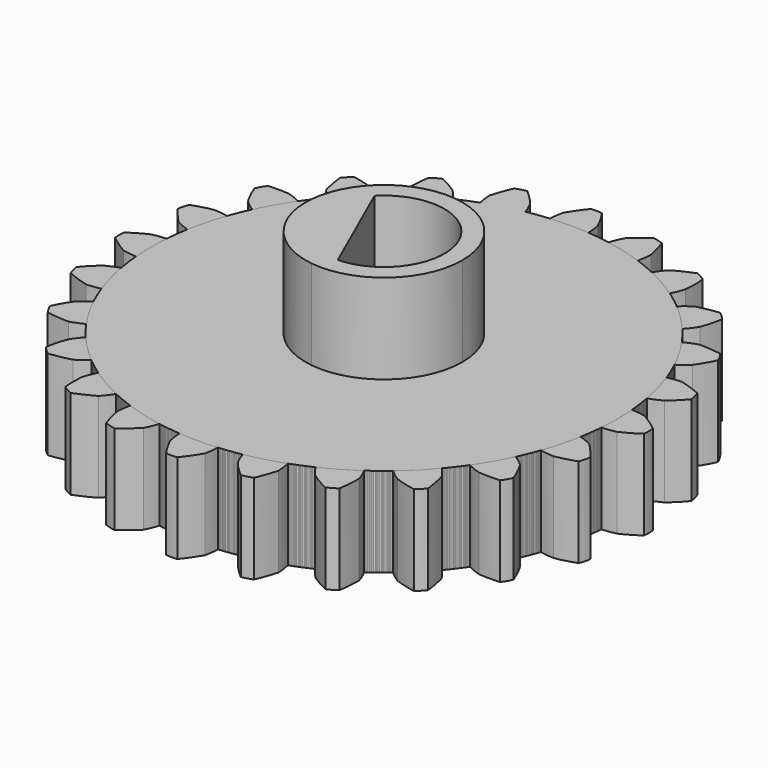
from build123d import *

# Parameters (mm, degrees)
F1_DEPTH = 5
F2_COUNT = 24
F4_DEPTH = 25
F6_DEPTH = 5


# Not quite as in the source:
# - a feature names something its author has since deleted; it is built from what else it names


with BuildPart() as f1:
    # F0 (on Top) → F1 (new body)
    with BuildSketch(Plane.XY):
        with BuildLine():
            ThreePointArc((-1.0909404477, 13.2232983115), (-8.7845379641, -9.3037195236), (13.009999547, 0.2700002324))
            ThreePointArc((13.009999547, 0.2700002324), (9.5634676777, 9.0865328091), (1.0513462123, 13.2282253085))
            ThreePointArc((1.0513462123, 13.2282253085), (-0.0198987816, 13.2699658512), (-1.0909404477, 13.2232983115))
        make_face()
        with BuildLine():
            ThreePointArc((-1.0909404477, 13.2232983115), (-0.0198987816, 13.2699658512), (1.0513462123, 13.2282253085))
            ThreePointArc((1.0513462123, 13.2282253085), (1.0154705709, 13.6241870699), (0.9417103543, 14.0148687927))
            ThreePointArc((0.9417103543, 14.0148687927), (0.6685218353, 14.5430546668), (0.3473408595, 15.0435095252))
            ThreePointArc((0.3473408595, 15.0435095252), (0.03481123, 15.0619613653), (-0.2776888118, 15.0430150292))
            ThreePointArc((-0.2776888118, 15.0430150292), (-0.6507511868, 14.5395305502), (-0.9878320882, 14.0112800205))
            ThreePointArc((-0.9878320882, 14.0112800205), (-1.0583416545, 13.6197695013), (-1.0909404477, 13.2232983115))
        make_face()
    extrude(amount=F1_DEPTH)


with BuildPart() as f2_1:
    # F2: instance of F1
    add(f1.part.rotate(Axis((0.009999547, 0.2700002324, 0), (0, 0, -1)), 1 * 360 / F2_COUNT))


with BuildPart() as f2_2:
    # F2: instance of F1
    add(f1.part.rotate(Axis((0.009999547, 0.2700002324, 0), (0, 0, -1)), 2 * 360 / F2_COUNT))


with BuildPart() as f2_3:
    # F2: instance of F1
    add(f1.part.rotate(Axis((0.009999547, 0.2700002324, 0), (0, 0, -1)), 3 * 360 / F2_COUNT))


with BuildPart() as f2_4:
    # F2: instance of F1
    add(f1.part.rotate(Axis((0.009999547, 0.2700002324, 0), (0, 0, -1)), 4 * 360 / F2_COUNT))


with BuildPart() as f2_5:
    # F2: instance of F1
    add(f1.part.rotate(Axis((0.009999547, 0.2700002324, 0), (0, 0, -1)), 5 * 360 / F2_COUNT))


with BuildPart() as f2_6:
    # F2: instance of F1
    add(f1.part.rotate(Axis((0.009999547, 0.2700002324, 0), (0, 0, -1)), 6 * 360 / F2_COUNT))


with BuildPart() as f2_7:
    # F2: instance of F1
    add(f1.part.rotate(Axis((0.009999547, 0.2700002324, 0), (0, 0, -1)), 7 * 360 / F2_COUNT))


with BuildPart() as f2_8:
    # F2: instance of F1
    add(f1.part.rotate(Axis((0.009999547, 0.2700002324, 0), (0, 0, -1)), 8 * 360 / F2_COUNT))


with BuildPart() as f2_9:
    # F2: instance of F1
    add(f1.part.rotate(Axis((0.009999547, 0.2700002324, 0), (0, 0, -1)), 9 * 360 / F2_COUNT))


with BuildPart() as f2_10:
    # F2: instance of F1
    add(f1.part.rotate(Axis((0.009999547, 0.2700002324, 0), (0, 0, -1)), 10 * 360 / F2_COUNT))


with BuildPart() as f2_11:
    # F2: instance of F1
    add(f1.part.rotate(Axis((0.009999547, 0.2700002324, 0), (0, 0, -1)), 11 * 360 / F2_COUNT))


with BuildPart() as f2_12:
    # F2: instance of F1
    add(f1.part.rotate(Axis((0.009999547, 0.2700002324, 0), (0, 0, -1)), 12 * 360 / F2_COUNT))


with BuildPart() as f2_13:
    # F2: instance of F1
    add(f1.part.rotate(Axis((0.009999547, 0.2700002324, 0), (0, 0, -1)), 13 * 360 / F2_COUNT))


with BuildPart() as f2_14:
    # F2: instance of F1
    add(f1.part.rotate(Axis((0.009999547, 0.2700002324, 0), (0, 0, -1)), 14 * 360 / F2_COUNT))


with BuildPart() as f2_15:
    # F2: instance of F1
    add(f1.part.rotate(Axis((0.009999547, 0.2700002324, 0), (0, 0, -1)), 15 * 360 / F2_COUNT))


with BuildPart() as f2_16:
    # F2: instance of F1
    add(f1.part.rotate(Axis((0.009999547, 0.2700002324, 0), (0, 0, -1)), 16 * 360 / F2_COUNT))


with BuildPart() as f2_17:
    # F2: instance of F1
    add(f1.part.rotate(Axis((0.009999547, 0.2700002324, 0), (0, 0, -1)), 17 * 360 / F2_COUNT))


with BuildPart() as f2_18:
    # F2: instance of F1
    add(f1.part.rotate(Axis((0.009999547, 0.2700002324, 0), (0, 0, -1)), 18 * 360 / F2_COUNT))


with BuildPart() as f2_19:
    # F2: instance of F1
    add(f1.part.rotate(Axis((0.009999547, 0.2700002324, 0), (0, 0, -1)), 19 * 360 / F2_COUNT))


with BuildPart() as f2_20:
    # F2: instance of F1
    add(f1.part.rotate(Axis((0.009999547, 0.2700002324, 0), (0, 0, -1)), 20 * 360 / F2_COUNT))


with BuildPart() as f2_21:
    # F2: instance of F1
    add(f1.part.rotate(Axis((0.009999547, 0.2700002324, 0), (0, 0, -1)), 21 * 360 / F2_COUNT))


with BuildPart() as f2_22:
    # F2: instance of F1
    add(f1.part.rotate(Axis((0.009999547, 0.2700002324, 0), (0, 0, -1)), 22 * 360 / F2_COUNT))


with BuildPart() as f2_23:
    # F2: instance of F1
    add(f1.part.rotate(Axis((0.009999547, 0.2700002324, 0), (0, 0, -1)), 23 * 360 / F2_COUNT))


with BuildPart() as f4_tool:
    # F3 (on face) → F4 (new body)
    with BuildSketch(Plane.XY.offset(5)):
        with BuildLine():
            ThreePointArc((0.133673408, -3.1189176238), (2.4512552702, -2.0837903178), (3.4011733055, 0.2700002324))
            ThreePointArc((3.4011733055, 0.2700002324), (2.404383524, 2.6714549646), (0, 3.661159248))
            ThreePointArc((0, 3.661159248), (-1.3078927109, 3.3946153217), (-2.4116129926, 2.6439952129))
            Line((-2.4116129926, 2.6439952129), (0.133673408, -3.1189176238))
        make_face()
    extrude(amount=-F4_DEPTH)


with BuildPart() as f1_1:
    add(f1.part)

    # F4: cut by f4_tool
    add(f4_tool.part, mode=Mode.SUBTRACT)


with BuildPart() as f2_1_1:
    add(f2_1.part)

    # F4: cut by f4_tool
    add(f4_tool.part, mode=Mode.SUBTRACT)


with BuildPart() as f2_2_1:
    add(f2_2.part)

    # F4: cut by f4_tool
    add(f4_tool.part, mode=Mode.SUBTRACT)


with BuildPart() as f2_3_1:
    add(f2_3.part)

    # F4: cut by f4_tool
    add(f4_tool.part, mode=Mode.SUBTRACT)


with BuildPart() as f2_4_1:
    add(f2_4.part)

    # F4: cut by f4_tool
    add(f4_tool.part, mode=Mode.SUBTRACT)


with BuildPart() as f2_5_1:
    add(f2_5.part)

    # F4: cut by f4_tool
    add(f4_tool.part, mode=Mode.SUBTRACT)


with BuildPart() as f2_6_1:
    add(f2_6.part)

    # F4: cut by f4_tool
    add(f4_tool.part, mode=Mode.SUBTRACT)


with BuildPart() as f2_7_1:
    add(f2_7.part)

    # F4: cut by f4_tool
    add(f4_tool.part, mode=Mode.SUBTRACT)


with BuildPart() as f2_8_1:
    add(f2_8.part)

    # F4: cut by f4_tool
    add(f4_tool.part, mode=Mode.SUBTRACT)


with BuildPart() as f2_9_1:
    add(f2_9.part)

    # F4: cut by f4_tool
    add(f4_tool.part, mode=Mode.SUBTRACT)


with BuildPart() as f2_10_1:
    add(f2_10.part)

    # F4: cut by f4_tool
    add(f4_tool.part, mode=Mode.SUBTRACT)


with BuildPart() as f2_11_1:
    add(f2_11.part)

    # F4: cut by f4_tool
    add(f4_tool.part, mode=Mode.SUBTRACT)


with BuildPart() as f2_12_1:
    add(f2_12.part)

    # F4: cut by f4_tool
    add(f4_tool.part, mode=Mode.SUBTRACT)


with BuildPart() as f2_13_1:
    add(f2_13.part)

    # F4: cut by f4_tool
    add(f4_tool.part, mode=Mode.SUBTRACT)


with BuildPart() as f2_14_1:
    add(f2_14.part)

    # F4: cut by f4_tool
    add(f4_tool.part, mode=Mode.SUBTRACT)


with BuildPart() as f2_15_1:
    add(f2_15.part)

    # F4: cut by f4_tool
    add(f4_tool.part, mode=Mode.SUBTRACT)


with BuildPart() as f2_16_1:
    add(f2_16.part)

    # F4: cut by f4_tool
    add(f4_tool.part, mode=Mode.SUBTRACT)


with BuildPart() as f2_17_1:
    add(f2_17.part)

    # F4: cut by f4_tool
    add(f4_tool.part, mode=Mode.SUBTRACT)


with BuildPart() as f2_18_1:
    add(f2_18.part)

    # F4: cut by f4_tool
    add(f4_tool.part, mode=Mode.SUBTRACT)


with BuildPart() as f2_19_1:
    add(f2_19.part)

    # F4: cut by f4_tool
    add(f4_tool.part, mode=Mode.SUBTRACT)


with BuildPart() as f2_20_1:
    add(f2_20.part)

    # F4: cut by f4_tool
    add(f4_tool.part, mode=Mode.SUBTRACT)


with BuildPart() as f2_21_1:
    add(f2_21.part)

    # F4: cut by f4_tool
    add(f4_tool.part, mode=Mode.SUBTRACT)


with BuildPart() as f2_22_1:
    add(f2_22.part)

    # F4: cut by f4_tool
    add(f4_tool.part, mode=Mode.SUBTRACT)


with BuildPart() as f2_23_1:
    add(f2_23.part)

    # F4: cut by f4_tool
    add(f4_tool.part, mode=Mode.SUBTRACT)


with BuildPart() as f6:
    # F5 (on face) → F6 (new body)
    with BuildSketch(Plane.XY.offset(5)):
        with BuildLine():
            ThreePointArc((-3.1464370209, 1.4647944375), (0.6173098397, 3.5899097505), (3.384999547, 0.2700002324))
            ThreePointArc((3.384999547, 0.2700002324), (1.9589480435, -2.4853989688), (-1.1140966058, -2.9122996968))
            Line((-1.1140966058, -2.9122996968), (-0.5787908965, -4.0651988188))
            ThreePointArc((-0.5787908965, -4.0651988188), (2.8879038896, -3.0251919616), (4.384999547, 0.2700002324))
            ThreePointArc((4.384999547, 0.2700002324), (1.2325486334, 4.4707143064), (-3.6817427302, 2.6176935595))
            Line((-3.6817427302, 2.6176935595), (-3.1464370209, 1.4647944375))
        make_face()
        with BuildLine():
            ThreePointArc((-1.1140966058, -2.9122996968), (-3.0511241614, -1.1513183954), (-3.1464370209, 1.4647944375))
            Line((-3.1464370209, 1.4647944375), (-3.6817427302, 2.6176935595))
            ThreePointArc((-3.6817427302, 2.6176935595), (-3.9581237787, -1.5724498406), (-0.5787908965, -4.0651988188))
            Line((-0.5787908965, -4.0651988188), (-1.1140966058, -2.9122996968))
        make_face()
        with BuildLine():
            Line((0.1266359476, -3.1029837507), (-2.4045755323, 2.6280613398))
            ThreePointArc((-2.4045755323, 2.6280613398), (-2.8355830234, 2.0847412153), (-3.1464370209, 1.4647944375))
            Line((-3.1464370209, 1.4647944375), (-1.1140966058, -2.9122996968))
            ThreePointArc((-1.1140966058, -2.9122996968), (-0.5026737312, -3.0658341625), (0.1266359476, -3.1029837507))
        make_face()
        with BuildLine():
            Line((-1.1140966058, -2.9122996968), (-3.1464370209, 1.4647944375))
            ThreePointArc((-3.1464370209, 1.4647944375), (-3.0511241614, -1.1513183954), (-1.1140966058, -2.9122996968))
        make_face()
    extrude(amount=F6_DEPTH)


solid = Compound([f1_1.part, f2_1_1.part, f2_2_1.part, f2_3_1.part, f2_4_1.part, f2_5_1.part, f2_6_1.part, f2_7_1.part, f2_8_1.part, f2_9_1.part, f2_10_1.part, f2_11_1.part, f2_12_1.part, f2_13_1.part, f2_14_1.part, f2_15_1.part, f2_16_1.part, f2_17_1.part, f2_18_1.part, f2_19_1.part, f2_20_1.part, f2_21_1.part, f2_22_1.part, f2_23_1.part, f6.part])
